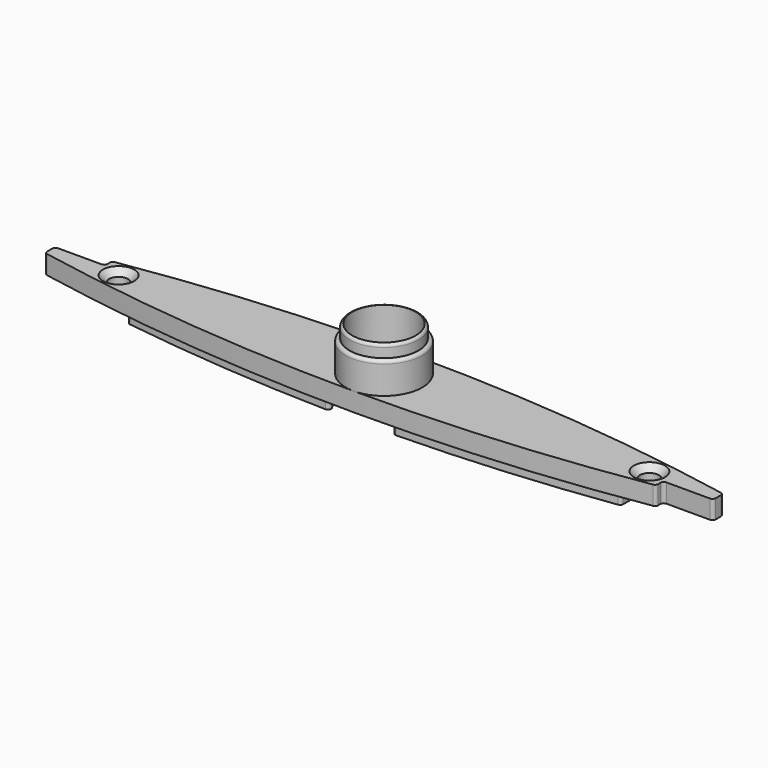
from build123d import *

# Parameters (mm, degrees)
F1_R      = 5.1
F2_DEPTH  = 3
F4_DEPTH  = 2
F7_R      = 6.125
F7_R_2    = 5.1
F8_DEPTH  = 5
F9_R      = 5.5
F9_R_2    = 5.1
F10_DEPTH = 2
F11_F1_R  = 0.5
F11_F2_R  = 0.5
F12_R     = 1.5
F13_DEPTH = 10.001
F14_SIZE  = 1


# Not quite as in the source:
# - a fillet or chamfer that OpenCascade refuses, or shapes differently, is made with other operations: its cross-section is extruded or revolved along the edge and cut away or added


with BuildPart() as f2:
    # F1 (on Top) → F2 (new body)
    with BuildSketch(Plane.XY):
        with BuildLine():
            Line((-53.5, 1), (-53.5, -1))
            ThreePointArc((-53.5, -1), (-4.0631867219, -6.095706229), (45.5, -2.4275662327))
            Line((45.5, -2.4275662327), (45.5, -1))
            Line((45.5, -1), (53.5, -1))
            Line((53.5, -1), (53.5, 1))
            ThreePointArc((53.5, 1), (4.0631867219, 6.095706229), (-45.5, 2.4275662327))
            Line((-45.5, 2.4275662327), (-45.5, 1))
            Line((-45.5, 1), (-53.5, 1))
        make_face()
        Circle(F1_R, mode=Mode.SUBTRACT)
    extrude(amount=F2_DEPTH)

    # F3 (on Top) → F4 (join)
    with BuildSketch(Plane.XY):
        with BuildLine():
            Line((-39.5, 1.9289369376), (-39.5, -1.9289369376))
            ThreePointArc((-39.5, -1.9289369376), (-22.0440441808, -3.8571649268), (-4.5016174848, -4.6888634039))
            ThreePointArc((-4.5016174848, -4.6888634039), (-6.5, 0), (-4.5016174848, 4.6888634039))
            ThreePointArc((-4.5016174848, 4.6888634039), (-22.0440441808, 3.8571649268), (-39.5, 1.9289369376))
        make_face()
        with BuildLine():
            Line((-38.5, -1.0597902373), (-38.5, 1.0597902373))
            ThreePointArc((-38.5, 1.0597902373), (-22.5636158392, 2.8124412347), (-6.5529405569, 3.6481461125))
            ThreePointArc((-6.5529405569, 3.6481461125), (-7.5, 0), (-6.5529405569, -3.6481461125))
            ThreePointArc((-6.5529405569, -3.6481461125), (-22.5636158392, -2.8124412347), (-38.5, -1.0597902373))
        make_face(mode=Mode.SUBTRACT)
        with BuildLine():
            ThreePointArc((4.5016174848, 4.6888634039), (6.5, 0), (4.5016174848, -4.6888634039))
            ThreePointArc((4.5016174848, -4.6888634039), (22.0440441808, -3.8571649268), (39.5, -1.9289369376))
            Line((39.5, -1.9289369376), (39.5, 1.9289369376))
            ThreePointArc((39.5, 1.9289369376), (22.0440441808, 3.8571649268), (4.5016174848, 4.6888634039))
        make_face()
        with BuildLine():
            ThreePointArc((6.5529405569, -3.6481461125), (7.5, 0), (6.5529405569, 3.6481461125))
            ThreePointArc((6.5529405569, 3.6481461125), (22.5636158392, 2.8124412347), (38.5, 1.0597902373))
            Line((38.5, 1.0597902373), (38.5, -1.0597902373))
            ThreePointArc((38.5, -1.0597902373), (22.5636158392, -2.8124412347), (6.5529405569, -3.6481461125))
        make_face(mode=Mode.SUBTRACT)
    extrude(amount=-F4_DEPTH)

    # F11: fillet of radius 0.5 on 16 edges, made by hand

    # F11_f1
    f11_f1_edges = [f2.edges().sort_by_distance(p)[0] for p in [
        (45.5, -1, 1.5),
        (-45.5, 1, 1.5),
    ]]
    fillet(f11_f1_edges, radius=F11_F1_R)

    # F11_f2
    f11_f2_edges = [f2.edges().sort_by_distance(p)[0] for p in [
        (53.5, -1, 1.5),
        (-45.5, 2.4275662327, 1.5),
        (-53.5, 1, 1.5),
        (-53.5, -1, 1.5),
        (-39.5, -1.9289369376, -1),
        (-39.5, 1.9289369376, -1),
        (39.5, 1.9289369376, -1),
        (39.5, -1.9289369376, -1),
        (4.5016174848, -4.6888634039, -1),
        (-4.5016174848, -4.6888634039, -1),
        (-4.5016174848, 4.6888634039, -1),
        (4.5016174848, 4.6888634039, -1),
        (53.5, 1, 1.5),
        (45.5, -2.4275662327, 1.5),
    ]]
    fillet(f11_f2_edges, radius=F11_F2_R)

    # F12 (on Top) → F13 (cut, through all)
    with BuildSketch(Plane.XY):
        with Locations((-42.5, 0)):
            Circle(F12_R)
        with Locations((42.5, 0)):
            Circle(F12_R)
    extrude(amount=F13_DEPTH, mode=Mode.SUBTRACT)

    # F14
    f14_edges = [f2.edges().sort_by_distance(p)[0] for p in [
        (-44, 0, 3),
        (41, 0, 3),
    ]]
    chamfer(f14_edges, length=F14_SIZE)


with BuildPart() as f8:
    # F7 (on face) → F8 (new body)
    with BuildSketch(Plane.XY.offset(3)):
        Circle(F7_R)
        Circle(F7_R_2, mode=Mode.SUBTRACT)
    extrude(amount=F8_DEPTH)

    # F9 (on face) → F10 (join)
    with BuildSketch(Plane.XY.offset(8)):
        Circle(F9_R)
        Circle(F9_R_2, mode=Mode.SUBTRACT)
    extrude(amount=F10_DEPTH)

    # F11#2: fillet of radius 0.5 on 2 edges, made by hand

    # F11_2_s1 → F11_2_t2 (revolve, cut)
    with BuildSketch(Plane.XZ):
        with BuildLine():
            ThreePointArc((6.125, 7.5), (5.9785533906, 7.8535533906), (5.625, 8))
            Line((5.625, 8), (6.125, 8))
            Line((6.125, 8), (6.125, 7.5))
        make_face()
    revolve(axis=Axis((0, 0, 8), (0, 0, 1)), mode=Mode.SUBTRACT)

    # F11_2_s3 → F11_2_t4 (revolve, cut)
    with BuildSketch(Plane.XZ):
        with BuildLine():
            ThreePointArc((5.5, 9.5101020514), (5.3872983346, 9.8263298175), (5.1, 10))
            Line((5.1, 10), (5.5, 10))
            Line((5.5, 10), (5.5, 9.5101020514))
        make_face()
    revolve(axis=Axis((0, 0, 10), (0, 0, 1)), mode=Mode.SUBTRACT)


solid = Compound([f2.part, f8.part])
